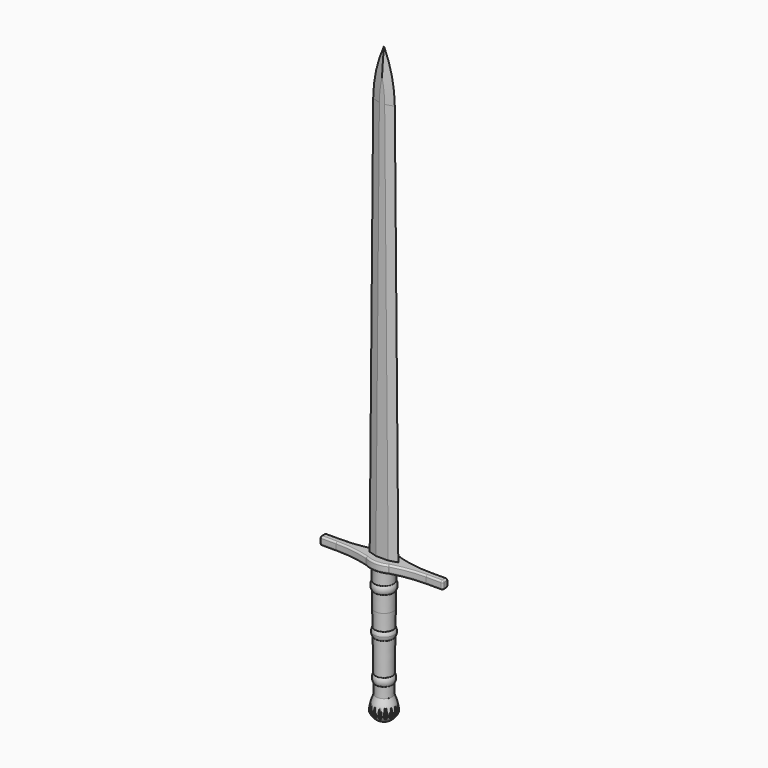
from build123d import *

# Parameters (mm, degrees)
F3_R        = 6.096
F4_DEPTH    = 5.08
F5_R        = 1.016
F9_DEPTH    = 25.4
F11_DEPTH   = 1.524
F12_SIZE2   = 5.08
F12_SIZE    = 1.524
F12_2_SIZE2 = 5.08
F12_2_SIZE  = 1.524
F13_SIZE2   = 5.07999
F13_SIZE    = 1.52399
F13_2_SIZE2 = 5.07999
F13_2_SIZE  = 1.52399
F15_DEPTH   = 1.016
F16_DEPTH   = 1.016


# Not quite as in the source:
# - a fillet or chamfer is up to 0.001 mm smaller than in the source, because OpenCascade refuses the exact size


with BuildPart() as f1:
    # F0 (on Right) → F1 (revolve)
    with BuildSketch(Plane.YZ):
        Polygon((0, -52.8828053154), (0, 0), (-6.096, 0), (-5.9849569233, -7.62), (-5.9125500429, -12.5887062471), (-5.7644496754, -22.7516523258), (-5.6170080735, -32.8693925764), (-5.5801451125, -35.399003345), (-5.5429509613, -37.9513410552), (-5.2477401821, -58.2093004428), (-5.1753333017, -63.17800669), (-5.08, -69.7199702263), (0, -69.7199702263), align=None)
    revolve(axis=Axis((0, 0, -26.4414026577), (0, 0, -1)))


with BuildPart() as f2:
    # F0 (on Right) → F2 (revolve)
    with BuildSketch(Plane.YZ):
        with BuildLine():
            Line((-5.5801451125, -35.399003345), (-5.6170080735, -32.8693925764))
            Line((-5.6170080735, -32.8693925764), (-5.6454416675, -32.9149807084))
            ThreePointArc((-5.6454416675, -32.9149807084), (-6.1733489014, -34.112499837), (-6.3433662141, -35.4101254473))
            Line((-6.3433662141, -35.4101254473), (-5.5801451125, -35.399003345))
        make_face()
        with BuildLine():
            Line((-5.5429509613, -37.9513410552), (-5.5801451125, -35.399003345))
            Line((-5.5801451125, -35.399003345), (-6.3433662141, -35.4101254473))
            ThreePointArc((-6.3433662141, -35.4101254473), (-6.1424234447, -36.7011342023), (-5.5872581617, -37.8838738655))
            Line((-5.5872581617, -37.8838738655), (-5.5429509613, -37.9513410552))
        make_face()
    revolve(axis=Axis((0, 0, -61.3013877708), (0, 0, -1)))


with BuildPart() as f2b:
    # F0 (on Right) → F2, piece 2 (revolve)
    with BuildSketch(Plane.YZ):
        with BuildLine():
            Line((-5.9125500429, -12.5887062471), (-5.9849569233, -7.62))
            ThreePointArc((-5.9849569233, -7.62), (-6.6757685355, -10.1149476102), (-5.9125500429, -12.5887062471))
        make_face()
    revolve(axis=Axis((0, 0, -61.3013877708), (0, 0, -1)))


with BuildPart() as f2c:
    # F0 (on Right) → F2, piece 3 (revolve)
    with BuildSketch(Plane.YZ):
        with BuildLine():
            ThreePointArc((-5.2477401821, -58.2093004428), (-5.9385517942, -60.704248053), (-5.1753333017, -63.17800669))
            Line((-5.1753333017, -63.17800669), (-5.2477401821, -58.2093004428))
        make_face()
    revolve(axis=Axis((0, 0, -61.3013877708), (0, 0, -1)))


with BuildPart() as f4:
    # F3 (on face) → F4 (new body)
    with BuildSketch(Plane.XY):
        with BuildLine():
            add(Edge.make_bspline(
                [(-7.0006083701, 5.0988825609), (-10.6986510224, 3.0821156927), (-10.6986510224, 0)],
                knots=[5.425705045, 5.425705045, 5.425705045, 6.2831853072, 6.2831853072, 6.2831853072], degree=2, weights=[1, 0.9094902307, 1]))
            ThreePointArc((-7.0006083701, 5.0988825609), (-17.3798265104, 2.8975491312), (-27.9641821004, 2.159))
            Line((-27.9641821004, 2.159), (-38.1151847541, 2.159))
            Line((-38.1151847541, 2.159), (-38.1151847541, 0))
            Line((-38.1151847541, 0), (-10.6986510224, 0))
        make_face()
        with BuildLine():
            add(Edge.make_bspline(
                [(-10.6986510224, 0), (-10.6986510224, -3.0821156927), (-7.0006083701, -5.0988825609)],
                knots=[0, 0, 0, 0.8574802622, 0.8574802622, 0.8574802622], degree=2, weights=[1, 0.9094902307, 1]))
            Line((-10.6986510224, 0), (-38.1151847541, 0))
            Line((-38.1151847541, 0), (-38.1151847541, -2.159))
            Line((-38.1151847541, -2.159), (-27.9641821004, -2.159))
            ThreePointArc((-27.9641821004, -2.159), (-17.3798265104, -2.8975491312), (-7.0006083701, -5.0988825609))
        make_face()
        with BuildLine():
            add(Edge.make_bspline(
                [(7.0006083701, 5.0988825609), (3.986233668, 6.7428038456), (0, 6.7428038456)],
                knots=[3.9990729158, 3.9990729158, 3.9990729158, 4.7123889804, 4.7123889804, 4.7123889804], degree=2, weights=[1, 0.9370688842, 1]))
            add(Edge.make_bspline(
                [(0, 6.7428038456), (-3.986233668, 6.7428038456), (-7.0006083701, 5.0988825609)],
                knots=[4.7123889804, 4.7123889804, 4.7123889804, 5.425705045, 5.425705045, 5.425705045], degree=2, weights=[1, 0.9370688842, 1]))
            add(Edge.make_bspline(
                [(-7.0006083701, 5.0988825609), (-10.6986510224, 3.0821156927), (-10.6986510224, 0)],
                knots=[5.425705045, 5.425705045, 5.425705045, 6.2831853072, 6.2831853072, 6.2831853072], degree=2, weights=[1, 0.9094902307, 1]))
            add(Edge.make_bspline(
                [(-10.6986510224, 0), (-10.6986510224, -3.0821156927), (-7.0006083701, -5.0988825609)],
                knots=[0, 0, 0, 0.8574802622, 0.8574802622, 0.8574802622], degree=2, weights=[1, 0.9094902307, 1]))
            add(Edge.make_bspline(
                [(-7.0006083701, -5.0988825609), (0, -8.9167387474), (7.0006083701, -5.0988825609)],
                knots=[0.8574802622, 0.8574802622, 0.8574802622, 2.2841123914, 2.2841123914, 2.2841123914], degree=2, weights=[1, 0.7561961875, 1]))
            add(Edge.make_bspline(
                [(7.0006083701, -5.0988825609), (16.3501695349, 0), (7.0006083701, 5.0988825609)],
                knots=[2.2841123914, 2.2841123914, 2.2841123914, 3.9990729158, 3.9990729158, 3.9990729158], degree=2, weights=[1, 0.6543449595, 1]))
        make_face()
        Circle(F3_R, mode=Mode.SUBTRACT)
        with BuildLine():
            ThreePointArc((27.9641821004, 2.159), (17.3798265104, 2.8975491312), (7.0006083701, 5.0988825609))
            add(Edge.make_bspline(
                [(7.0006083701, -5.0988825609), (16.3501695349, 0), (7.0006083701, 5.0988825609)],
                knots=[2.2841123914, 2.2841123914, 2.2841123914, 3.9990729158, 3.9990729158, 3.9990729158], degree=2, weights=[1, 0.6543449595, 1]))
            ThreePointArc((7.0006083701, -5.0988825609), (17.3798265104, -2.8975491312), (27.9641821004, -2.159))
            Line((27.9641821004, -2.159), (38.1151847541, -2.159))
            Line((38.1151847541, -2.159), (38.1151847541, 0))
            Line((38.1151847541, 0), (38.1151847541, 2.159))
            Line((38.1151847541, 2.159), (27.9641821004, 2.159))
        make_face()
        Circle(F3_R)
    extrude(amount=F4_DEPTH)

    # F5
    f5_edges = [f4.edges().sort_by_distance(p)[0] for p in [
        (-17.379827, -2.897549, 5.08),
        (-33.039683, -2.159, 5.08),
        (-33.039683, -2.159, 0),
        (-17.379827, -2.897549, 0),
        (-17.379827, 2.897549, 0),
        (-17.379827, 2.897549, 5.08),
        (-33.039683, 2.159, 5.08),
        (-38.115185, -2.159, 2.54),
        (-38.115185, 2.159, 2.54),
        (-38.115185, 0, 0),
        (-38.115185, 0, 5.08),
        (17.379827, -2.897549, 5.08),
        (17.379827, -2.897549, 0),
        (17.379827, 2.897549, 5.08),
        (17.379827, 2.897549, 0),
        (38.115185, -2.159, 2.54),
        (38.115185, 2.159, 2.54),
        (38.115185, 0, 0),
        (38.115185, 0, 5.08),
        (-7.000608, -5.098883, 2.54),
        (7.000608, -5.098883, 2.54),
        (0, -6.742804, 0),
        (0, -6.742804, 5.08),
        (7.000608, 5.098883, 2.54),
        (-7.000608, 5.098883, 2.54),
        (0, 6.742804, 0),
        (0, 6.742804, 5.08),
        (-33.039683, 2.159, 0),
        (33.039683, 2.159, 0),
        (33.039683, 2.159, 5.08),
        (33.039683, -2.159, 0),
        (33.039683, -2.159, 5.08),
    ]]
    fillet(f5_edges, radius=F5_R)


with BuildPart() as f7:
    # F6 (on Front) → F7 (revolve)
    with BuildSketch(Plane.XZ):
        with BuildLine():
            Line((0, -69.7199702263), (-5.08, -69.7199702263))
            ThreePointArc((-5.08, -69.7199702263), (-6.561531353, -74.0620145214), (-7.3748384602, -78.5771906376))
            ThreePointArc((-7.3748384602, -78.5771906376), (-4.5876194941, -82.5227172308), (0, -84.035832243))
            Line((0, -84.035832243), (0, -75.643517077))
            Line((0, -75.643517077), (0, -72.6817436516))
            Line((0, -72.6817436516), (0, -69.7199702263))
        make_face()
    revolve(axis=Axis((0, 0, -78.3587879473), (0, 0, -1)))

    # F8 (on face) → F9 (cut)
    with BuildSketch(Plane.XY.offset(-69.7199702263)):
        with BuildLine():
            Line((-5.9628928688, 2.8529602326), (-6.4203100442, 3.6287547797))
            ThreePointArc((-6.4203100442, 3.6287547797), (-6.813462309, 2.8222284951), (-7.1057618816, 1.9739276575))
            Line((-7.1057618816, 1.9739276575), (-6.23374951, 2.1990544561))
            Line((-6.23374951, 2.1990544561), (-5.9628928688, 2.8529602326))
        make_face()
        with BuildLine():
            Line((-6.6007752903, 0.3538912561), (-7.3202573765, 0.895585985))
            ThreePointArc((-7.3202573765, 0.895585985), (-7.3748384602, 0), (-7.3202573765, -0.895585985))
            Line((-7.3202573765, -0.895585985), (-6.6007752903, -0.3538912561))
            Line((-6.6007752903, -0.3538912561), (-6.6007752903, 0.3538912561))
        make_face()
        with BuildLine():
            ThreePointArc((-7.1057618816, -1.9739276575), (-6.813462309, -2.8222284951), (-6.4203100442, -3.6287547797))
            Line((-6.4203100442, -3.6287547797), (-5.9628928688, -2.8529602326))
            Line((-5.9628928688, -2.8529602326), (-6.23374951, -2.1990544561))
            Line((-6.23374951, -2.1990544561), (-7.1057618816, -1.9739276575))
        make_face()
        with BuildLine():
            ThreePointArc((-5.809478554, -4.5429287079), (-5.2147982854, -5.2147982854), (-4.5429287079, -5.809478554))
            Line((-4.5429287079, -5.809478554), (-4.4172140618, -4.9176918759))
            Line((-4.4172140618, -4.9176918759), (-4.9176918759, -4.4172140618))
            Line((-4.9176918759, -4.4172140618), (-5.809478554, -4.5429287079))
        make_face()
        with BuildLine():
            ThreePointArc((-3.6287547797, -6.4203100442), (-2.8222284951, -6.813462309), (-1.9739276575, -7.1057618816))
            Line((-1.9739276575, -7.1057618816), (-2.1990544561, -6.23374951))
            Line((-2.1990544561, -6.23374951), (-2.8529602326, -5.9628928688))
            Line((-2.8529602326, -5.9628928688), (-3.6287547797, -6.4203100442))
        make_face()
        with BuildLine():
            ThreePointArc((-0.895585985, -7.3202573765), (0, -7.3748384602), (0.895585985, -7.3202573765))
            Line((0.895585985, -7.3202573765), (0.3538912561, -6.6007752903))
            Line((0.3538912561, -6.6007752903), (-0.3538912561, -6.6007752903))
            Line((-0.3538912561, -6.6007752903), (-0.895585985, -7.3202573765))
        make_face()
        with BuildLine():
            ThreePointArc((1.9739276575, -7.1057618816), (2.8222284951, -6.813462309), (3.6287547797, -6.4203100442))
            Line((3.6287547797, -6.4203100442), (2.8529602326, -5.9628928688))
            Line((2.8529602326, -5.9628928688), (2.1990544561, -6.23374951))
            Line((2.1990544561, -6.23374951), (1.9739276575, -7.1057618816))
        make_face()
        with BuildLine():
            ThreePointArc((4.5429287079, -5.809478554), (5.2147982854, -5.2147982854), (5.809478554, -4.5429287079))
            Line((5.809478554, -4.5429287079), (4.9176918759, -4.4172140618))
            Line((4.9176918759, -4.4172140618), (4.4172140618, -4.9176918759))
            Line((4.4172140618, -4.9176918759), (4.5429287079, -5.809478554))
        make_face()
        with BuildLine():
            ThreePointArc((6.4203100442, -3.6287547797), (6.813462309, -2.8222284951), (7.1057618816, -1.9739276575))
            Line((7.1057618816, -1.9739276575), (6.23374951, -2.1990544561))
            Line((6.23374951, -2.1990544561), (5.9628928688, -2.8529602326))
            Line((5.9628928688, -2.8529602326), (6.4203100442, -3.6287547797))
        make_face()
        with BuildLine():
            ThreePointArc((7.3202573765, -0.895585985), (7.3611805423, -0.4486238266), (7.3748384602, 0))
            ThreePointArc((7.3748384602, 0), (7.3611805423, 0.4486238266), (7.3202573765, 0.895585985))
            Line((7.3202573765, 0.895585985), (6.6007752903, 0.3538912561))
            Line((6.6007752903, 0.3538912561), (6.6007752903, -0.3538912561))
            Line((6.6007752903, -0.3538912561), (7.3202573765, -0.895585985))
        make_face()
        with BuildLine():
            Line((6.23374951, 2.1990544561), (7.1057618816, 1.9739276575))
            ThreePointArc((7.1057618816, 1.9739276575), (6.813462309, 2.8222284951), (6.4203100442, 3.6287547797))
            Line((6.4203100442, 3.6287547797), (5.9628928688, 2.8529602326))
            Line((5.9628928688, 2.8529602326), (6.23374951, 2.1990544561))
        make_face()
        with BuildLine():
            Line((4.9176918759, 4.4172140618), (5.809478554, 4.5429287079))
            ThreePointArc((5.809478554, 4.5429287079), (5.2147982854, 5.2147982854), (4.5429287079, 5.809478554))
            Line((4.5429287079, 5.809478554), (4.4172140618, 4.9176918759))
            Line((4.4172140618, 4.9176918759), (4.9176918759, 4.4172140618))
        make_face()
        with BuildLine():
            Line((2.8529602326, 5.9628928688), (3.6287547797, 6.4203100442))
            ThreePointArc((3.6287547797, 6.4203100442), (2.8222284951, 6.813462309), (1.9739276575, 7.1057618816))
            Line((1.9739276575, 7.1057618816), (2.1990544561, 6.23374951))
            Line((2.1990544561, 6.23374951), (2.8529602326, 5.9628928688))
        make_face()
        with BuildLine():
            Line((0.3538912561, 6.6007752903), (0.895585985, 7.3202573765))
            ThreePointArc((0.895585985, 7.3202573765), (0, 7.3748384602), (-0.895585985, 7.3202573765))
            Line((-0.895585985, 7.3202573765), (-0.3538912561, 6.6007752903))
            Line((-0.3538912561, 6.6007752903), (0.3538912561, 6.6007752903))
        make_face()
        with BuildLine():
            Line((-2.1990544561, 6.23374951), (-1.9739276575, 7.1057618816))
            ThreePointArc((-1.9739276575, 7.1057618816), (-2.8222284951, 6.813462309), (-3.6287547797, 6.4203100442))
            Line((-3.6287547797, 6.4203100442), (-2.8529602326, 5.9628928688))
            Line((-2.8529602326, 5.9628928688), (-2.1990544561, 6.23374951))
        make_face()
        with BuildLine():
            Line((-4.4172140618, 4.9176918759), (-4.5429287079, 5.809478554))
            ThreePointArc((-4.5429287079, 5.809478554), (-5.2147982854, 5.2147982854), (-5.809478554, 4.5429287079))
            Line((-5.809478554, 4.5429287079), (-4.9176918759, 4.4172140618))
            Line((-4.9176918759, 4.4172140618), (-4.4172140618, 4.9176918759))
        make_face()
    extrude(amount=-F9_DEPTH, mode=Mode.SUBTRACT)


with BuildPart() as f11:
    # F10 (on Front) → F11 (new body, symmetric)
    with BuildSketch(Plane.XZ):
        with BuildLine():
            Line((-6.8294036171, 5.08), (-6.4298777883, 5.08))
            add(Edge.make_bspline(
                [(-6.4298777883, 5.08), (-4.2865851922, 5.08), (-2.1432925961, 5.08), (0, 5.08)],
                knots=[0, 0, 0, 0, 0.5, 0.5, 0.5, 0.5], degree=3))
            Line((0, 5.08), (0, 284.48))
            ThreePointArc((0, 284.48), (-4.9524226532, 269.4709338522), (-6.7197585285, 253.7650406693))
            Line((-6.7197585285, 253.7650406693), (-8.89, 5.08))
            Line((-8.89, 5.08), (-6.8294036171, 5.08))
        make_face()
        with BuildLine():
            Line((0, 284.48), (0, 5.08))
            add(Edge.make_bspline(
                [(0, 5.08), (2.1432925961, 5.08), (4.2865851922, 5.08), (6.4298777883, 5.08)],
                knots=[0.5, 0.5, 0.5, 0.5, 1, 1, 1, 1], degree=3))
            Line((6.4298777883, 5.08), (6.8294036171, 5.08))
            Line((6.8294036171, 5.08), (8.89, 5.08))
            Line((8.89, 5.08), (6.7197585285, 253.7650406693))
            ThreePointArc((6.7197585285, 253.7650406693), (4.9524226532, 269.4709338522), (0, 284.48))
        make_face()
    extrude(amount=F11_DEPTH, both=True)

    # F12
    f12_edges = [f11.edges().sort_by_distance(p)[0] for p in [
        (-7.804879, -1.524, 129.42252),
    ]]
    f12_side = f11.faces().sort_by_distance((-7.804879, 0, 129.42252))[0]
    chamfer(f12_edges, length=F12_SIZE, length2=F12_SIZE2, reference=f12_side)

    # F12#2
    f12_2_edges = [f11.edges().sort_by_distance(p)[0] for p in [
        (7.804879, -1.524, 129.42252),
    ]]
    f12_2_side = f11.faces().sort_by_distance((7.804879, 0, 129.42252))[0]
    chamfer(f12_2_edges, length=F12_2_SIZE, length2=F12_2_SIZE2, reference=f12_2_side)

    # F13 (size 1.524 and 5.08 in the source; OpenCascade refuses exactly that, so slightly less here)
    f13_edges = [f11.edges().sort_by_distance(p)[0] for p in [
        (7.804879, 1.524, 129.42252),
    ]]
    f13_side = f11.faces().sort_by_distance((7.804879, 0.762, 129.42252))[0]
    chamfer(f13_edges, length=F13_SIZE, length2=F13_SIZE2, reference=f13_side)

    # F13#2 (size 1.524 and 5.08 in the source; OpenCascade refuses exactly that, so slightly less here)
    f13_2_edges = [f11.edges().sort_by_distance(p)[0] for p in [
        (-7.804879, 1.524, 129.42252),
    ]]
    f13_2_side = f11.faces().sort_by_distance((-7.804879, 0.762, 129.42252))[0]
    chamfer(f13_2_edges, length=F13_2_SIZE, length2=F13_2_SIZE2, reference=f13_2_side)

    # F14 (on Front) → F16 (join, symmetric)
    with BuildSketch(Plane.XZ):
        with BuildLine():
            add(Edge.make_bspline(
                [(-3.8098065618, 5.08), (-2.5398710412, 5.08), (-1.2699355206, 5.08), (0, 5.08)],
                knots=[0.2037419149, 0.2037419149, 0.2037419149, 0.2037419149, 0.5, 0.5, 0.5, 0.5], degree=3))
            Line((-3.8098065618, 5.08), (-5.5546094663, 5.08))
            Line((-5.5546094663, 5.08), (-3.5690569784, -75.1555636525))
            Line((-3.5690569784, -75.1555636525), (0, -75.1555636525))
            Line((0, -75.1555636525), (0, 5.08))
        make_face()
        with BuildLine():
            add(Edge.make_bspline(
                [(0, 5.08), (1.2699355206, 5.08), (2.5398710412, 5.08), (3.8098065618, 5.08)],
                knots=[0.5, 0.5, 0.5, 0.5, 0.7962580851, 0.7962580851, 0.7962580851, 0.7962580851], degree=3))
            Line((0, 5.08), (0, -75.1555636525))
            Line((0, -75.1555636525), (3.5690569784, -75.1555636525))
            Line((3.5690569784, -75.1555636525), (5.5546094663, 5.08))
            add(Edge.make_bspline(
                [(3.8098065618, 5.08), (4.39140753, 5.08), (4.9730084982, 5.08), (5.5546094663, 5.08)],
                knots=[0.7962580851, 0.7962580851, 0.7962580851, 0.7962580851, 0.9319374061, 0.9319374061, 0.9319374061, 0.9319374061], degree=3))
        make_face()
    extrude(amount=F16_DEPTH, both=True)


with BuildPart() as f15_tool:
    # F14 (on Front) → F15 (new body, symmetric)
    with BuildSketch(Plane.XZ):
        with BuildLine():
            add(Edge.make_bspline(
                [(-3.8098065618, 5.08), (-2.5398710412, 5.08), (-1.2699355206, 5.08), (0, 5.08)],
                knots=[0.2037419149, 0.2037419149, 0.2037419149, 0.2037419149, 0.5, 0.5, 0.5, 0.5], degree=3))
            Line((-3.8098065618, 5.08), (-5.5546094663, 5.08))
            Line((-5.5546094663, 5.08), (-3.5690569784, -75.1555636525))
            Line((-3.5690569784, -75.1555636525), (0, -75.1555636525))
            Line((0, -75.1555636525), (0, 5.08))
        make_face()
        with BuildLine():
            add(Edge.make_bspline(
                [(0, 5.08), (1.2699355206, 5.08), (2.5398710412, 5.08), (3.8098065618, 5.08)],
                knots=[0.5, 0.5, 0.5, 0.5, 0.7962580851, 0.7962580851, 0.7962580851, 0.7962580851], degree=3))
            Line((0, 5.08), (0, -75.1555636525))
            Line((0, -75.1555636525), (3.5690569784, -75.1555636525))
            Line((3.5690569784, -75.1555636525), (5.5546094663, 5.08))
            add(Edge.make_bspline(
                [(3.8098065618, 5.08), (4.39140753, 5.08), (4.9730084982, 5.08), (5.5546094663, 5.08)],
                knots=[0.7962580851, 0.7962580851, 0.7962580851, 0.7962580851, 0.9319374061, 0.9319374061, 0.9319374061, 0.9319374061], degree=3))
        make_face()
    extrude(amount=F15_DEPTH, both=True)


with BuildPart() as f1_1:
    add(f1.part)

    # F15: cut by f15_tool
    add(f15_tool.part, mode=Mode.SUBTRACT)


with BuildPart() as f4_1:
    add(f4.part)

    # F15: cut by f15_tool
    add(f15_tool.part, mode=Mode.SUBTRACT)


with BuildPart() as f7_1:
    add(f7.part)

    # F15: cut by f15_tool
    add(f15_tool.part, mode=Mode.SUBTRACT)


solid = Compound([f2.part, f2b.part, f2c.part, f11.part, f1_1.part, f4_1.part, f7_1.part])
